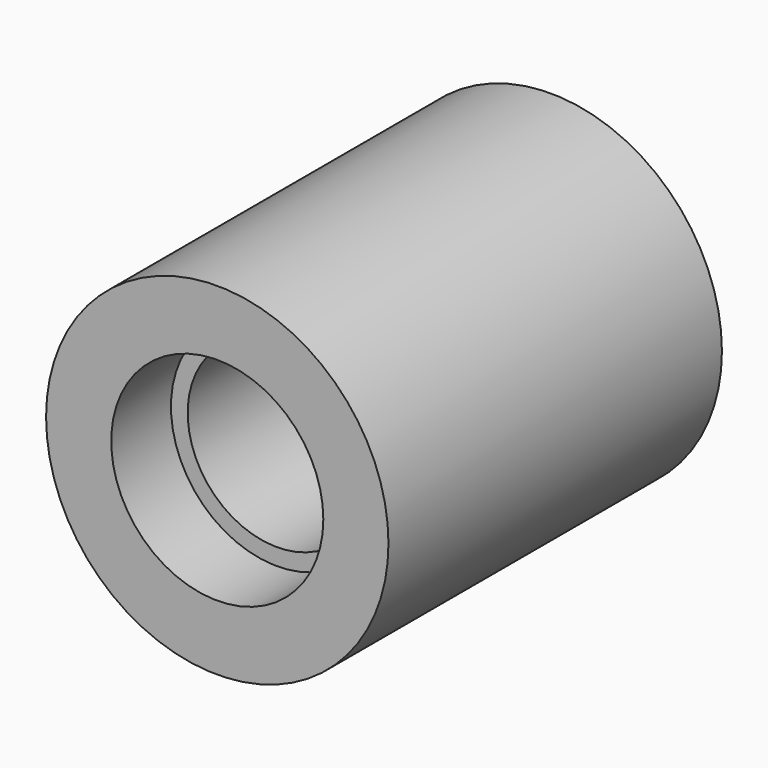
from build123d import *

# Parameters (mm, degrees)
F0_R     = 36.5125
F1_DEPTH = 88.9
F2_R     = 19.05
F3_DEPTH = 88.901
F4_R     = 22.6187
F5_DEPTH = 15.9258


# Not quite as in the source:
# - a pattern or mirror of a feature is missing from the dataset's text; its kind, count and spacing are read off the source's solid


with BuildPart() as f1:
    # F0 (on Front) → F1 (new body)
    with BuildSketch(Plane.XZ):
        Circle(F0_R)
    extrude(amount=F1_DEPTH)

    # F2 (on Front) → F3 (cut, through all)
    with BuildSketch(Plane.XZ):
        Circle(F2_R)
    extrude(amount=F3_DEPTH, mode=Mode.SUBTRACT)

    # F4 (on Front) → F5 (cut)
    with BuildSketch(Plane.XZ):
        Circle(F4_R)
    f5 = extrude(amount=F5_DEPTH, mode=Mode.SUBTRACT)

    # F5_copies: F5 across plane
    add(f5.mirror(Plane(origin=(0, -44.45, 0), x_dir=(0, 0, -1), z_dir=(0, -1, 0))), mode=Mode.SUBTRACT)


solid = f1.part
